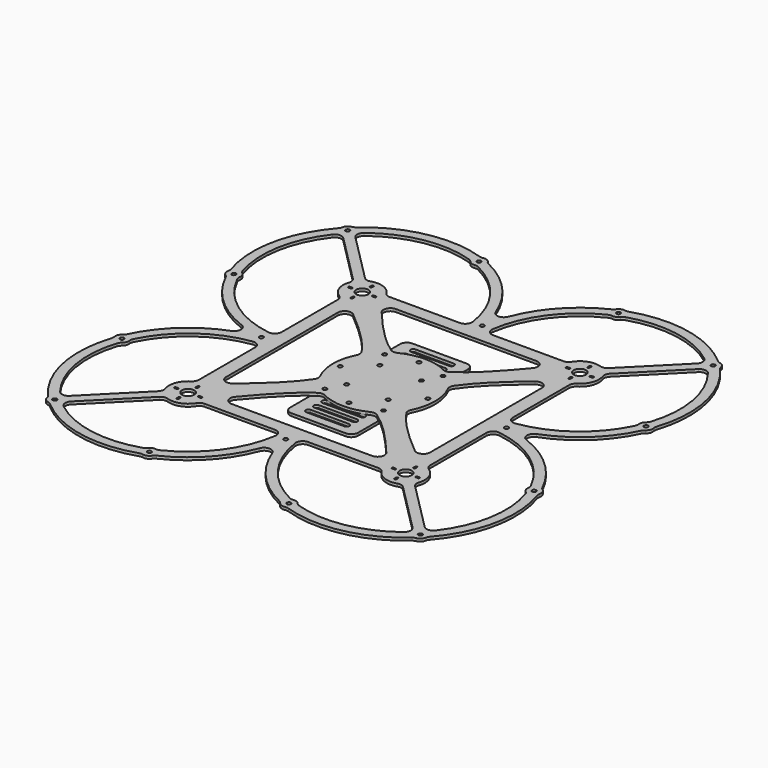
from build123d import *

# Parameters (mm, degrees)
F0_R     = 1.5
F0_R_2   = 4.5
F1_DEPTH = 2
F3_DEPTH = 2
F4_D     = 3
F4_DEPTH = 2.001
F5_D     = 3


with BuildPart() as f1:
    # F0 (on Top) → F1 (new body)
    with BuildSketch(Plane.XY):
        with BuildLine():
            ThreePointArc((-4.6783625728, -108.4060017489), (3e-10, -105.1703496836), (4.6783625734, -108.4060017489))
            ThreePointArc((4.6783625734, -108.4060017489), (20.6623898885, -134.3994303853), (45.1726415046, -152.5762020239))
            ThreePointArc((45.1726415046, -152.5762020239), (46.2648777579, -153.2890175874), (47.1356036045, -154.2600595848))
            ThreePointArc((47.1356036044, -154.2600595849), (49.3956359115, -156.0747849076), (52.2827571645, -156.3307241522))
            ThreePointArc((52.2827571645, -156.3307241521), (53.5833623617, -156.2331937381), (54.8649423602, -156.4753481681))
            ThreePointArc((54.8649423602, -156.4753481681), (96.0251691017, -158.888807541), (132.9814512388, -140.6070608478))
            ThreePointArc((132.9814512388, -140.6070608478), (134.0669737734, -139.8840623088), (135.3025491662, -139.4664027472))
            ThreePointArc((135.3025491663, -139.4664027473), (137.8609824083, -138.1042744963), (139.2338336739, -135.5515791701))
            ThreePointArc((139.2338336738, -135.55157917), (139.6566739459, -134.317767124), (140.3842208964, -133.235287796))
            ThreePointArc((140.3842208964, -133.235287796), (158.8415006809, -96.2563147842), (156.517113249, -54.992373563))
            ThreePointArc((156.517113249, -54.992373563), (156.2770940729, -53.7103919501), (156.3767909625, -52.4099510284))
            ThreePointArc((156.3767909626, -52.4099510283), (156.1256615791, -49.5224074254), (154.3147036453, -47.2593551971))
            ThreePointArc((154.3147036452, -47.2593551972), (153.3451134923, -46.3870129501), (152.6341184177, -45.2935907697))
            ThreePointArc((152.6341184177, -45.2935907697), (134.4488352599, -20.7077210859), (108.4060017484, -4.6783625732))
            ThreePointArc((108.4060017484, -4.6783625732), (105.1703496824, -2e-10), (108.4060017477, 4.6783625732))
            ThreePointArc((108.4060017484, 4.6783625735), (134.4488352601, 20.7077210863), (152.634118418, 45.2935907703))
            ThreePointArc((152.634118418, 45.2935907703), (153.3451134926, 46.3870129507), (154.3147036455, 47.2593551978))
            ThreePointArc((154.3147036455, 47.2593551978), (156.1256615793, 49.5224074261), (156.3767909627, 52.409951029))
            ThreePointArc((156.3767909627, 52.409951029), (156.2770940731, 53.7103919508), (156.5171132493, 54.9923735636))
            ThreePointArc((156.5171132493, 54.9923735636), (158.8415006809, 96.256314785), (140.3842208962, 133.2352877967))
            ThreePointArc((140.3842208962, 133.2352877967), (139.6566739457, 134.3177671247), (139.2338336737, 135.5515791707))
            ThreePointArc((139.2338336737, 135.5515791707), (137.8609824081, 138.1042744969), (135.3025491661, 139.4664027479))
            ThreePointArc((135.3025491661, 139.4664027479), (134.0669737732, 139.8840623095), (132.9814512386, 140.6070608485))
            ThreePointArc((132.9814512386, 140.6070608485), (96.0251691014, 158.8888075416), (54.8649423599, 156.4753481684))
            ThreePointArc((54.8649423599, 156.4753481684), (53.5833623613, 156.2331937384), (52.2827571641, 156.3307241524))
            ThreePointArc((52.2827571641, 156.3307241524), (49.3956359112, 156.0747849078), (47.1356036041, 154.2600595851))
            ThreePointArc((47.1356036041, 154.2600595851), (46.2648777575, 153.2890175877), (45.1726415042, 152.5762020242))
            ThreePointArc((45.1726415042, 152.5762020242), (20.6623898881, 134.3994303854), (4.6783625731, 108.4060017488))
            ThreePointArc((4.6783625731, 108.4060017488), (0, 105.1703496833), (-4.6783625732, 108.4060017486))
            ThreePointArc((-4.6783625731, 108.4060017484), (-20.6623898882, 134.3994303851), (-45.1726415045, 152.576202024))
            ThreePointArc((-45.1726415045, 152.576202024), (-46.2648777578, 153.2890175875), (-47.1356036044, 154.2600595849))
            ThreePointArc((-47.1356036044, 154.2600595849), (-49.3956359115, 156.0747849076), (-52.2827571644, 156.3307241522))
            ThreePointArc((-52.2827571644, 156.3307241522), (-53.5833623617, 156.2331937382), (-54.8649423602, 156.4753481682))
            ThreePointArc((-54.8649423602, 156.4753481682), (-96.0251691017, 158.8888075411), (-132.9814512389, 140.6070608479))
            ThreePointArc((-132.9814512389, 140.6070608479), (-134.0669737735, 139.8840623089), (-135.3025491663, 139.4664027473))
            ThreePointArc((-135.3025491663, 139.4664027473), (-137.8609824083, 138.1042744963), (-139.2338336739, 135.5515791701))
            ThreePointArc((-139.2338336739, 135.5515791701), (-139.656673946, 134.317767124), (-140.3842208964, 133.2352877961))
            ThreePointArc((-140.3842208964, 133.2352877961), (-158.841500681, 96.2563147843), (-156.5171132492, 54.9923735629))
            ThreePointArc((-156.5171132492, 54.9923735629), (-156.277094073, 53.7103919501), (-156.3767909626, 52.4099510283))
            ThreePointArc((-156.3767909626, 52.4099510283), (-156.1256615791, 49.5224074254), (-154.3147036453, 47.2593551971))
            ThreePointArc((-154.3147036453, 47.2593551971), (-153.3451134924, 46.38701295), (-152.6341184178, 45.2935907696))
            ThreePointArc((-152.6341184178, 45.2935907696), (-134.44883526, 20.7077210858), (-108.4060017484, 4.6783625731))
            ThreePointArc((-108.4060017484, 4.6783625731), (-105.1703496831, 0), (-108.4060017484, -4.6783625731))
            ThreePointArc((-108.4060017484, -4.6783625731), (-134.4488352601, -20.7077210859), (-152.6341184181, -45.2935907699))
            ThreePointArc((-152.6341184181, -45.2935907699), (-153.3451134927, -46.3870129503), (-154.3147036456, -47.2593551973))
            ThreePointArc((-154.3147036453, -47.2593551971), (-156.1256615791, -49.5224074254), (-156.3767909626, -52.4099510283))
            ThreePointArc((-156.3767909629, -52.4099510286), (-156.2770940733, -53.7103919503), (-156.5171132495, -54.9923735632))
            ThreePointArc((-156.5171132495, -54.9923735632), (-158.8415006814, -96.2563147847), (-140.3842208967, -133.2352877966))
            ThreePointArc((-140.3842208967, -133.2352877966), (-139.6566739462, -134.3177671246), (-139.2338336742, -135.5515791707))
            ThreePointArc((-139.2338336739, -135.5515791701), (-137.8609824083, -138.1042744963), (-135.3025491663, -139.4664027473))
            ThreePointArc((-135.3025491665, -139.4664027479), (-134.0669737737, -139.8840623095), (-132.9814512391, -140.6070608485))
            ThreePointArc((-132.9814512391, -140.6070608485), (-96.0251691018, -158.8888075418), (-54.8649423601, -156.4753481689))
            ThreePointArc((-54.8649423601, -156.4753481689), (-53.5833623616, -156.2331937389), (-52.2827571643, -156.3307241529))
            ThreePointArc((-52.2827571644, -156.3307241522), (-49.3956359115, -156.0747849076), (-47.1356036044, -154.2600595849))
            ThreePointArc((-47.1356036043, -154.2600595856), (-46.2648777577, -153.2890175882), (-45.1726415044, -152.5762020247))
            ThreePointArc((-45.1726415044, -152.5762020247), (-20.662389888, -134.3994303857), (-4.6783625728, -108.4060017489))
        make_face()
        with Locations((-134.3328737249, -134.5613309295)):
            Circle(F0_R, mode=Mode.SUBTRACT)
        with Locations((-51.261755673, -151.4360785108)):
            Circle(F0_R, mode=Mode.SUBTRACT)
        with BuildLine():
            Line((-63.8445055783, -85.0000000006), (-12.2338580112, -85.0000000003))
            ThreePointArc((-12.2338580112, -85.0000000003), (-8.4490439447, -86.7327102241), (-7.2874242894, -90.7299270076))
            ThreePointArc((-7.2874242894, -90.7299270076), (-20.659248064, -123.3696340744), (-47.697444438, -146.0211701219))
            ThreePointArc((-47.697444438, -146.0211701219), (-49.1034491785, -146.4668977043), (-50.578326435, -146.4830062853))
            ThreePointArc((-50.5783264353, -146.4830062847), (-53.1278754345, -146.797372114), (-55.1848415227, -148.3361757032))
            ThreePointArc((-55.1848415226, -148.3361757039), (-56.2599847867, -149.345922885), (-57.5829585673, -149.9980446406))
            ThreePointArc((-57.5829585673, -149.9980446406), (-92.7749506491, -152.3812865043), (-125.0248290937, -138.0948772713))
            ThreePointArc((-125.0248290937, -138.0948772713), (-126.9516515101, -134.4630557491), (-125.504859117, -130.6147361204))
            Line((-125.504859117, -130.6147361204), (-89.5414765934, -94.5001358666))
            ThreePointArc((-89.5414765934, -94.5001358666), (-87.1537232514, -93.1635209665), (-84.4199717038, -93.2839696686))
            ThreePointArc((-84.4199717038, -93.2839696686), (-75.230169782, -93.1623979469), (-68.0959514787, -87.3684210532))
            ThreePointArc((-68.0959514787, -87.3684210532), (-66.2778268953, -85.6320545604), (-63.8445055783, -85.0000000006))
        make_face(mode=Mode.SUBTRACT)
        with BuildLine():
            ThreePointArc((-79.2499999996, -89.4999999999), (-79.9999999996, -90.2499999999), (-80.7499999996, -89.4999999999))
            Line((-80.7499999996, -89.4999999999), (-80.7499999996, -87.9999999999))
            ThreePointArc((-80.7499999996, -87.9999999999), (-79.9999999996, -87.2499999999), (-79.2499999996, -87.9999999999))
            Line((-79.2499999996, -87.9999999999), (-79.2499999996, -89.4999999999))
        make_face(mode=Mode.SUBTRACT)
        with Locations((-151.4838529462, -51.3807972166)):
            Circle(F0_R, mode=Mode.SUBTRACT)
        with BuildLine():
            ThreePointArc((-85.0000000002, -63.8445055787), (-85.63205456, -66.2778268956), (-87.3684210528, -68.095951479))
            ThreePointArc((-87.3684210528, -68.095951479), (-93.164159415, -75.2350333787), (-93.2806998405, -84.4297868752))
            ThreePointArc((-93.2806998405, -84.4297868752), (-93.156247777, -87.1550368598), (-94.4808633594, -89.5399622996))
            Line((-94.4808633594, -89.5399622996), (-130.4597965629, -125.6701786202))
            ThreePointArc((-130.4597965629, -125.6701786202), (-134.3041683835, -127.1329757672), (-137.9445459786, -125.2181334358))
            ThreePointArc((-137.9445459785, -125.2181334359), (-152.3491388585, -92.9557750247), (-150.035290906, -57.6995957941))
            ThreePointArc((-150.035290906, -57.6995957941), (-149.3853739289, -56.3755375132), (-148.3774191744, -55.2987136553))
            ThreePointArc((-148.3774191741, -55.2987136551), (-146.8420443134, -53.2391870077), (-146.5319260821, -50.6891178603))
            ThreePointArc((-146.5319260824, -50.6891178605), (-146.5182744455, -49.214215816), (-146.0748896721, -47.8074705118))
            ThreePointArc((-146.0748896721, -47.8074705118), (-123.419045392, -20.6953922764), (-90.7299270074, -7.2874242898))
            ThreePointArc((-90.7299270074, -7.2874242898), (-86.7327102239, -8.4490439451), (-85.0000000001, -12.2338580116))
            Line((-85.0000000001, -12.2338580116), (-85.0000000002, -63.8445055787))
        make_face(mode=Mode.SUBTRACT)
        with BuildLine():
            ThreePointArc((-87.9999999996, -79.2499999999), (-87.2499999996, -79.9999999999), (-87.9999999996, -80.7499999999))
            Line((-87.9999999996, -80.7499999999), (-89.4999999996, -80.75))
            ThreePointArc((-89.4999999996, -80.75), (-90.2499999996, -80), (-89.4999999996, -79.25))
            Line((-89.4999999996, -79.25), (-87.9999999996, -79.2499999999))
        make_face(mode=Mode.SUBTRACT)
        with Locations((-80, -80.0000000004)):
            Circle(F0_R_2, mode=Mode.SUBTRACT)
        with BuildLine():
            ThreePointArc((-71.9999999996, -80.7499999998), (-72.7499999996, -79.9999999998), (-71.9999999996, -79.2499999998))
            Line((-71.9999999996, -79.2499999998), (-70.4999999996, -79.2499999998))
            ThreePointArc((-70.4999999996, -79.2499999998), (-69.7499999996, -79.9999999998), (-70.4999999996, -80.7499999998))
            Line((-70.4999999996, -80.7499999998), (-71.9999999996, -80.7499999998))
        make_face(mode=Mode.SUBTRACT)
        with BuildLine():
            ThreePointArc((-79.2499999997, -71.9999999999), (-79.9999999997, -72.7499999999), (-80.7499999997, -71.9999999999))
            Line((-80.7499999997, -71.9999999999), (-80.7499999997, -70.4999999999))
            ThreePointArc((-80.7499999997, -70.4999999999), (-79.9999999997, -69.7499999999), (-79.2499999997, -70.4999999999))
            Line((-79.2499999997, -70.4999999999), (-79.2499999997, -71.9999999999))
        make_face(mode=Mode.SUBTRACT)
        with Locations((51.261755673, -151.4360785108)):
            Circle(F0_R, mode=Mode.SUBTRACT)
        with Locations((4e-10, -90.3351748412)):
            Circle(F0_R, mode=Mode.SUBTRACT)
        with BuildLine():
            Line((12.2338580118, -85.0000000002), (63.8445055786, -85))
            ThreePointArc((63.8445055786, -85), (66.2778268956, -85.6320545598), (68.095951479, -87.3684210526))
            ThreePointArc((68.095951479, -87.3684210526), (75.230169782, -93.1623979461), (84.4199717034, -93.283969668))
            ThreePointArc((84.4199717034, -93.283969668), (87.1537232509, -93.1635209659), (89.5414765929, -94.500135866))
            Line((89.5414765929, -94.500135866), (125.5048591164, -130.6147361197))
            ThreePointArc((125.5048591164, -130.6147361197), (126.9516515096, -134.4630557483), (125.0248290934, -138.0948772705))
            ThreePointArc((125.0248290934, -138.0948772705), (92.774950649, -152.3812865033), (57.5829585674, -149.9980446396))
            ThreePointArc((57.5829585674, -149.9980446396), (56.2599847868, -149.3459228841), (55.1848415227, -148.336175703))
            ThreePointArc((55.1848415227, -148.3361757032), (53.1278754345, -146.797372114), (50.5783264353, -146.4830062847))
            ThreePointArc((50.5783264354, -146.4830062845), (49.1034491789, -146.4668977035), (47.6974444384, -146.021170121))
            ThreePointArc((47.6974444384, -146.021170121), (20.6592480646, -123.3696340739), (7.2874242901, -90.7299270075))
            ThreePointArc((7.2874242901, -90.7299270075), (8.4490439453, -86.732710224), (12.2338580118, -85.0000000002))
        make_face(mode=Mode.SUBTRACT)
        with BuildLine():
            Line((79.2500000004, -89.4999999995), (79.2500000004, -87.9999999995))
            ThreePointArc((79.2500000004, -87.9999999995), (80.0000000004, -87.2499999995), (80.7500000004, -87.9999999995))
            Line((80.7500000004, -87.9999999995), (80.7500000004, -89.4999999995))
            ThreePointArc((80.7500000004, -89.4999999995), (80.0000000004, -90.2499999995), (79.2500000004, -89.4999999995))
        make_face(mode=Mode.SUBTRACT)
        with Locations((134.3328737249, -134.5613309295)):
            Circle(F0_R, mode=Mode.SUBTRACT)
        with BuildLine():
            add(Edge.make_bspline(
                [(-21.8118215176, -33.8721360964), (-14.5412143451, -28.9488980864), (-7.2706071343, -25.9999999845), (7.65e-08, -26)],
                knots=[0.3347589279, 0.3347589279, 0.3347589279, 0.3347589279, 0.5, 0.5, 0.5, 0.5], degree=3))
            add(Edge.make_bspline(
                [(7.65e-08, -26), (7.2706072364, -26.0000000155), (14.5412143964, -28.948898107), (21.8118215577, -33.8721361171)],
                knots=[0.5, 0.5, 0.5, 0.5, 0.6652410721, 0.6652410721, 0.6652410721, 0.6652410721], degree=3))
            add(Edge.make_bspline(
                [(21.8118215178, -33.8721360963), (33.0610814435, -41.4894894667), (44.3103413693, -53.8332210309), (55.5596012951, -67.2936601505)],
                knots=[0.6652410721, 0.6652410721, 0.6652410721, 0.6652410721, 0.9209060704, 0.9209060704, 0.9209060704, 0.9209060704], degree=3))
            ThreePointArc((55.5596012951, -67.2936601505), (56.2524587842, -72.6175812561), (51.7230162552, -75.5))
            Line((51.7230162552, -75.5), (-51.7230162547, -75.5000000003))
            ThreePointArc((-51.7230162547, -75.5000000003), (-56.2524587837, -72.6175812564), (-55.5596012947, -67.2936601507))
            add(Edge.make_bspline(
                [(-55.5596012947, -67.2936601507), (-44.310341369, -53.8332210311), (-33.0610814433, -41.4894894668), (-21.8118215176, -33.8721360964)],
                knots=[0.0790939296, 0.0790939296, 0.0790939296, 0.0790939296, 0.3347589279, 0.3347589279, 0.3347589279, 0.3347589279], degree=3))
        make_face(mode=Mode.SUBTRACT)
        with BuildLine():
            Line((70.5000000004, -79.2499999995), (72.0000000004, -79.2499999995))
            ThreePointArc((72.0000000004, -79.2499999995), (72.7500000004, -79.9999999995), (72.0000000004, -80.7499999995))
            Line((72.0000000004, -80.7499999995), (70.5000000004, -80.7499999995))
            ThreePointArc((70.5000000004, -80.7499999995), (69.7500000004, -79.9999999995), (70.5000000004, -79.2499999995))
        make_face(mode=Mode.SUBTRACT)
        with Locations((80, -80)):
            Circle(F0_R_2, mode=Mode.SUBTRACT)
        with BuildLine():
            ThreePointArc((80.7500000004, -71.9999999995), (80.0000000004, -72.7499999995), (79.2500000004, -71.9999999995))
            Line((79.2500000004, -71.9999999995), (79.2500000004, -70.4999999995))
            ThreePointArc((79.2500000004, -70.4999999995), (80.0000000004, -69.7499999995), (80.7500000004, -70.4999999995))
            Line((80.7500000004, -70.4999999995), (80.7500000004, -71.9999999995))
        make_face(mode=Mode.SUBTRACT)
        with BuildLine():
            add(Edge.make_bspline(
                [(33.8663150036, -21.8197185294), (28.9467838534, -14.548575325), (25.9999990678, -7.2776728311), (25.9999990322, -0.0072165863)],
                knots=[0.3346551775, 0.3346551775, 0.3346551775, 0.3346551775, 0.4998909766, 0.4998909766, 0.4998909766, 0.4998909766], degree=3))
            add(Edge.make_bspline(
                [(25.9999990322, -0.0072165863), (25.9999990322, -0.0048110575), (26.0009742814, 7.2678904272), (28.9508771882, 14.540145319), (33.87301354, 21.8097056412)],
                knots=[0.4998909766, 0.4998909766, 0.4998909766, 0.4998909766, 0.4999456471, 0.6651778067, 0.6651778067, 0.6651778067, 0.6651778067], degree=3))
            add(Edge.make_bspline(
                [(33.87301354, 21.8097056412), (41.3952497644, 32.9193836512), (53.5259879584, 44.0283862504), (66.7895824295, 55.137274203)],
                knots=[0.6651778067, 0.6651778067, 0.6651778067, 0.6651778067, 0.9176932284, 0.9176932284, 0.9176932284, 0.9176932284], degree=3))
            ThreePointArc((66.7895824295, 55.137274203), (72.1151851744, 55.8346983966), (75.0000273883, 51.3041211152))
            Line((75.0000273883, 51.3041211152), (74.9999753624, -51.3429242195))
            ThreePointArc((74.9999753624, -51.3429242195), (72.1142737789, -55.8738975411), (66.7880804223, -55.1748573441))
            add(Edge.make_bspline(
                [(66.7880804223, -55.1748573441), (53.5232646354, -44.0564048176), (41.3886054554, -32.9377802776), (33.8663150036, -21.8197185294)],
                knots=[0.0819986465, 0.0819986465, 0.0819986465, 0.0819986465, 0.3346551775, 0.3346551775, 0.3346551775, 0.3346551775], degree=3))
        make_face(mode=Mode.SUBTRACT)
        with BuildLine():
            Line((88.0000000004, -79.2499999995), (89.5000000004, -79.2499999995))
            ThreePointArc((89.5000000004, -79.2499999995), (90.2500000004, -79.9999999995), (89.5000000004, -80.7499999995))
            Line((89.5000000004, -80.7499999995), (88.0000000004, -80.7499999995))
            ThreePointArc((88.0000000004, -80.7499999995), (87.2500000004, -79.9999999995), (88.0000000004, -79.2499999995))
        make_face(mode=Mode.SUBTRACT)
        with BuildLine():
            ThreePointArc((87.3684210526, -68.095951479), (85.6320545598, -66.2778268956), (85, -63.8445055786))
            Line((85, -63.8445055786), (85, -12.2338580112))
            ThreePointArc((85, -12.2338580112), (86.7327102238, -8.4490439446), (90.7299270073, -7.2874242894))
            ThreePointArc((90.7299270073, -7.2874242894), (123.4190453919, -20.6953922759), (146.0748896721, -47.8074705114))
            ThreePointArc((146.0748896721, -47.8074705114), (146.5182744455, -49.2142158156), (146.5319260824, -50.6891178601))
            ThreePointArc((146.5319260821, -50.6891178603), (146.8420443134, -53.2391870077), (148.3774191741, -55.298713655))
            ThreePointArc((148.3774191744, -55.2987136549), (149.3853739289, -56.3755375129), (150.035290906, -57.6995957937))
            ThreePointArc((150.035290906, -57.6995957937), (152.3491388585, -92.9557750243), (137.9445459785, -125.2181334356))
            ThreePointArc((137.9445459785, -125.2181334356), (134.3041683835, -127.132975767), (130.4597965628, -125.67017862))
            Line((130.4597965628, -125.67017862), (94.4808633591, -89.5399622991))
            ThreePointArc((94.4808633591, -89.5399622991), (93.1562477767, -87.1550368593), (93.2806998402, -84.4297868747))
            ThreePointArc((93.2806998402, -84.4297868747), (93.1641594147, -75.2350333784), (87.3684210526, -68.095951479))
        make_face(mode=Mode.SUBTRACT)
        with Locations((151.4838529462, -51.3807972166)):
            Circle(F0_R, mode=Mode.SUBTRACT)
        with Locations((-90.0851748436, 0)):
            Circle(F0_R, mode=Mode.SUBTRACT)
        with Locations((-151.4838529462, 51.3807972166)):
            Circle(F0_R, mode=Mode.SUBTRACT)
        with BuildLine():
            Line((-85, 63.8445055786), (-85, 12.2338580115))
            ThreePointArc((-85, 12.2338580115), (-86.7327102238, 8.449043945), (-90.7299270073, 7.2874242898))
            ThreePointArc((-90.7299270073, 7.2874242898), (-123.4190453917, 20.6953922762), (-146.0748896718, 47.8074705116))
            ThreePointArc((-146.0748896718, 47.8074705116), (-146.5182744452, 49.2142158157), (-146.5319260821, 50.6891178603))
            ThreePointArc((-146.5319260821, 50.6891178603), (-146.8420443134, 53.2391870077), (-148.3774191741, 55.2987136551))
            ThreePointArc((-148.3774191741, 55.2987136551), (-149.3853739286, 56.375537513), (-150.0352909057, 57.6995957938))
            ThreePointArc((-150.0352909057, 57.6995957938), (-152.3491388582, 92.9557750243), (-137.9445459782, 125.2181334353))
            ThreePointArc((-137.9445459782, 125.2181334353), (-134.3041683832, 127.1329757667), (-130.4597965625, 125.6701786198))
            Line((-130.4597965625, 125.6701786198), (-94.4808633591, 89.5399622991))
            ThreePointArc((-94.4808633591, 89.5399622991), (-93.1562477767, 87.1550368593), (-93.2806998402, 84.4297868747))
            ThreePointArc((-93.2806998402, 84.4297868747), (-93.1641594147, 75.2350333784), (-87.3684210526, 68.095951479))
            ThreePointArc((-87.3684210526, 68.095951479), (-85.6320545598, 66.2778268956), (-85, 63.8445055786))
        make_face(mode=Mode.SUBTRACT)
        with BuildLine():
            Line((-89.5, 80.75), (-88, 80.75))
            ThreePointArc((-88, 80.75), (-87.25, 80), (-88, 79.25))
            Line((-88, 79.25), (-89.5, 79.25))
            ThreePointArc((-89.5, 79.25), (-90.25, 80), (-89.5, 80.75))
        make_face(mode=Mode.SUBTRACT)
        with BuildLine():
            add(Edge.make_bspline(
                [(-33.8721360963, 21.8118215178), (-28.9488980863, 14.5412143452), (-26.0000000096, 7.2706071963), (-26, 4.74e-08)],
                knots=[0.3347589279, 0.3347589279, 0.3347589279, 0.3347589279, 0.5, 0.5, 0.5, 0.5], degree=3))
            add(Edge.make_bspline(
                [(-26, 4.74e-08), (-25.9999999904, -7.2706071331), (-28.9488980734, -14.5412143135), (-33.8721360834, -21.811821493)],
                knots=[0.5, 0.5, 0.5, 0.5, 0.6652410721, 0.6652410721, 0.6652410721, 0.6652410721], degree=3))
            add(Edge.make_bspline(
                [(-33.8721360963, -21.8118215178), (-41.3943179444, -32.9205327334), (-53.5255126569, -44.029243949), (-66.7896643299, -55.1379551646)],
                knots=[0.6652410721, 0.6652410721, 0.6652410721, 0.6652410721, 0.9177117815, 0.9177117815, 0.9177117815, 0.9177117815], degree=3))
            ThreePointArc((-66.7896643299, -55.1379551646), (-72.1152212253, -55.835258214), (-75.0000000043, -51.3047130828))
            Line((-75.0000000043, -51.3047130828), (-75.000000004, 51.3047130826))
            ThreePointArc((-75.000000004, 51.3047130826), (-72.1152212251, 55.8352582138), (-66.7896643296, 55.1379551644))
            add(Edge.make_bspline(
                [(-66.7896643296, 55.1379551644), (-53.5255126568, 44.0292439489), (-41.3943179444, 32.9205327333), (-33.8721360963, 21.8118215178)],
                knots=[0.0822882185, 0.0822882185, 0.0822882185, 0.0822882185, 0.3347589279, 0.3347589279, 0.3347589279, 0.3347589279], degree=3))
        make_face(mode=Mode.SUBTRACT)
        with BuildLine():
            Line((-80.75, 70.5), (-80.75, 72))
            ThreePointArc((-80.75, 72), (-80, 72.75), (-79.25, 72))
            Line((-79.25, 72), (-79.25, 70.5))
            ThreePointArc((-79.25, 70.5), (-80, 69.75), (-80.75, 70.5))
        make_face(mode=Mode.SUBTRACT)
        with Locations((-80, 80)):
            Circle(F0_R_2, mode=Mode.SUBTRACT)
        with BuildLine():
            Line((-70.5, 79.25), (-72, 79.25))
            ThreePointArc((-72, 79.25), (-72.75, 80), (-72, 80.75))
            Line((-72, 80.75), (-70.5, 80.75))
            ThreePointArc((-70.5, 80.75), (-69.75, 80), (-70.5, 79.25))
        make_face(mode=Mode.SUBTRACT)
        with Locations((-134.3328737249, 134.5613309295)):
            Circle(F0_R, mode=Mode.SUBTRACT)
        with BuildLine():
            Line((-79.25, 89.5), (-79.25, 88))
            ThreePointArc((-79.25, 88), (-80, 87.25), (-80.75, 88))
            Line((-80.75, 88), (-80.75, 89.5))
            ThreePointArc((-80.75, 89.5), (-80, 90.25), (-79.25, 89.5))
        make_face(mode=Mode.SUBTRACT)
        with BuildLine():
            ThreePointArc((-63.8445055786, 85), (-66.2778268956, 85.6320545598), (-68.095951479, 87.3684210527))
            ThreePointArc((-68.095951479, 87.3684210527), (-75.2301697821, 93.1623979461), (-84.4199717034, 93.283969668))
            ThreePointArc((-84.4199717034, 93.283969668), (-87.153723251, 93.1635209659), (-89.5414765929, 94.500135866))
            Line((-89.5414765929, 94.500135866), (-125.5048591166, 130.6147361199))
            ThreePointArc((-125.5048591166, 130.6147361199), (-126.9516515098, 134.4630557485), (-125.0248290936, 138.0948772707))
            ThreePointArc((-125.0248290936, 138.0948772707), (-92.774950649, 152.3812865036), (-57.5829585674, 149.9980446399))
            ThreePointArc((-57.5829585674, 149.9980446399), (-56.2599847868, 149.3459228844), (-55.1848415227, 148.3361757032))
            ThreePointArc((-55.1848415227, 148.3361757032), (-53.1278754345, 146.797372114), (-50.5783264353, 146.4830062847))
            ThreePointArc((-50.5783264353, 146.4830062847), (-49.1034491788, 146.4668977038), (-47.6974444383, 146.0211701213))
            ThreePointArc((-47.6974444383, 146.0211701213), (-20.6592480643, 123.369634074), (-7.2874242898, 90.7299270073))
            ThreePointArc((-7.2874242898, 90.7299270073), (-8.4490439451, 86.7327102239), (-12.2338580115, 85.0000000002))
            Line((-12.2338580115, 85.0000000002), (-63.8445055786, 85))
        make_face(mode=Mode.SUBTRACT)
        with Locations((-51.261755673, 151.4360785108)):
            Circle(F0_R, mode=Mode.SUBTRACT)
        Polygon((26, -0.0072165863), (26, -26), (1.147e-07, -26), (-26, -26), (-26, 7.1e-08), (-26, 26), (-7.1e-08, 26), (26, 26), align=None, mode=Mode.SUBTRACT)
        with BuildLine():
            add(Edge.make_bspline(
                [(-4.74e-08, 26), (7.2706071331, 25.9999999904), (14.5412143135, 28.9488980734), (21.811821493, 33.8721360834)],
                knots=[0.5, 0.5, 0.5, 0.5, 0.6652410721, 0.6652410721, 0.6652410721, 0.6652410721], degree=3))
            add(Edge.make_bspline(
                [(-21.8118215178, 33.8721360963), (-14.5412143452, 28.9488980863), (-7.2706071963, 26.0000000096), (-4.74e-08, 26)],
                knots=[0.3347589279, 0.3347589279, 0.3347589279, 0.3347589279, 0.5, 0.5, 0.5, 0.5], degree=3))
            add(Edge.make_bspline(
                [(-55.5596012951, 67.2936601505), (-44.3103413693, 53.8332210308), (-33.0610814435, 41.4894894667), (-21.8118215178, 33.8721360963)],
                knots=[0.0790939296, 0.0790939296, 0.0790939296, 0.0790939296, 0.3347589279, 0.3347589279, 0.3347589279, 0.3347589279], degree=3))
            ThreePointArc((-55.5596012951, 67.2936601505), (-56.2524587842, 72.6175812561), (-51.7230162551, 75.5))
            Line((-51.7230162551, 75.5), (51.7230162553, 75.5000000003))
            ThreePointArc((51.7230162553, 75.5000000003), (56.2524587844, 72.6175812564), (55.5596012953, 67.2936601507))
            add(Edge.make_bspline(
                [(21.8118215178, 33.8721360963), (33.0610814436, 41.4894894667), (44.3103413695, 53.833221031), (55.5596012953, 67.2936601507)],
                knots=[0.6652410721, 0.6652410721, 0.6652410721, 0.6652410721, 0.9209060704, 0.9209060704, 0.9209060704, 0.9209060704], degree=3))
        make_face(mode=Mode.SUBTRACT)
        with BuildLine():
            ThreePointArc((79.25, 72.0000000004), (80, 72.7500000004), (80.75, 72.0000000004))
            Line((80.75, 72.0000000004), (80.75, 70.5000000004))
            ThreePointArc((80.75, 70.5000000004), (80, 69.7500000004), (79.25, 70.5000000004))
            Line((79.25, 70.5000000004), (79.25, 72.0000000004))
        make_face(mode=Mode.SUBTRACT)
        with BuildLine():
            ThreePointArc((72, 80.7500000003), (72.75, 80.0000000003), (72, 79.2500000003))
            Line((72, 79.2500000003), (70.5, 79.2500000003))
            ThreePointArc((70.5, 79.2500000003), (69.75, 80.0000000003), (70.5, 80.7500000003))
            Line((70.5, 80.7500000003), (72, 80.7500000003))
        make_face(mode=Mode.SUBTRACT)
        with Locations((80, 80.0000000004)):
            Circle(F0_R_2, mode=Mode.SUBTRACT)
        with Locations((90.085174844, 5e-10)):
            Circle(F0_R, mode=Mode.SUBTRACT)
        with BuildLine():
            ThreePointArc((89.5, 80.7500000004), (90.25, 80.0000000004), (89.5, 79.2500000004))
            Line((89.5, 79.2500000004), (88, 79.2500000004))
            ThreePointArc((88, 79.2500000004), (87.25, 80.0000000004), (88, 80.7500000004))
            Line((88, 80.7500000004), (89.5, 80.7500000004))
        make_face(mode=Mode.SUBTRACT)
        with BuildLine():
            ThreePointArc((85, 63.844505579), (85.6320545598, 66.2778268959), (87.3684210526, 68.0959514793))
            ThreePointArc((87.3684210526, 68.0959514793), (93.1641594147, 75.2350333788), (93.2806998401, 84.4297868751))
            ThreePointArc((93.2806998401, 84.4297868751), (93.1562477767, 87.1550368597), (94.4808633591, 89.5399622995))
            Line((94.4808633591, 89.5399622995), (130.4597965625, 125.6701786201))
            ThreePointArc((130.4597965625, 125.6701786201), (134.3041683832, 127.1329757671), (137.9445459782, 125.2181334357))
            ThreePointArc((137.9445459782, 125.2181334357), (152.3491388582, 92.9557750248), (150.0352909058, 57.6995957945))
            ThreePointArc((150.0352909058, 57.6995957945), (149.3853739287, 56.3755375137), (148.3774191742, 55.2987136557))
            ThreePointArc((148.3774191742, 55.2987136557), (146.8420443135, 53.2391870084), (146.5319260822, 50.6891178609))
            ThreePointArc((146.5319260822, 50.6891178609), (146.5182744454, 49.2142158164), (146.0748896719, 47.8074705122))
            ThreePointArc((146.0748896719, 47.8074705122), (123.4190453919, 20.6953922767), (90.7299270073, 7.2874242901))
            ThreePointArc((90.7299270073, 7.2874242901), (86.7327102238, 8.4490439454), (85, 12.2338580119))
            Line((85, 12.2338580119), (85, 63.844505579))
        make_face(mode=Mode.SUBTRACT)
        with Locations((151.4838529464, 51.3807972172)):
            Circle(F0_R, mode=Mode.SUBTRACT)
        with Locations((0, 90.3351748417)):
            Circle(F0_R, mode=Mode.SUBTRACT)
        with BuildLine():
            ThreePointArc((80.75, 88.0000000004), (80, 87.2500000004), (79.25, 88.0000000004))
            Line((79.25, 88.0000000004), (79.25, 89.5000000004))
            ThreePointArc((79.25, 89.5000000004), (80, 90.2500000004), (80.75, 89.5000000004))
            Line((80.75, 89.5000000004), (80.75, 88.0000000004))
        make_face(mode=Mode.SUBTRACT)
        with BuildLine():
            ThreePointArc((68.095951479, 87.368421053), (66.2778268956, 85.6320545602), (63.8445055786, 85.0000000003))
            Line((63.8445055786, 85.0000000003), (12.2338580115, 85.0000000002))
            ThreePointArc((12.2338580115, 85.0000000002), (8.4490439449, 86.732710224), (7.2874242898, 90.7299270077))
            ThreePointArc((7.2874242898, 90.7299270077), (20.6592480642, 123.3696340742), (47.697444438, 146.0211701215))
            ThreePointArc((47.697444438, 146.0211701215), (49.1034491785, 146.466897704), (50.578326435, 146.4830062849))
            ThreePointArc((50.578326435, 146.4830062849), (53.1278754342, 146.7973721143), (55.1848415223, 148.3361757035))
            ThreePointArc((55.1848415223, 148.3361757035), (56.2599847865, 149.3459228846), (57.582958567, 149.9980446401))
            ThreePointArc((57.582958567, 149.9980446401), (92.7749506489, 152.381286504), (125.0248290935, 138.0948772711))
            ThreePointArc((125.0248290935, 138.0948772711), (126.9516515098, 134.4630557488), (125.5048591166, 130.6147361202))
            Line((125.5048591166, 130.6147361202), (89.5414765929, 94.5001358664))
            ThreePointArc((89.5414765929, 94.5001358664), (87.1537232509, 93.1635209663), (84.4199717034, 93.2839696684))
            ThreePointArc((84.4199717034, 93.2839696684), (75.230169782, 93.1623979465), (68.095951479, 87.368421053))
        make_face(mode=Mode.SUBTRACT)
        with Locations((51.2617556727, 151.436078511)):
            Circle(F0_R, mode=Mode.SUBTRACT)
        with Locations((134.3328737246, 134.5613309301)):
            Circle(F0_R, mode=Mode.SUBTRACT)
        Polygon((1.147e-07, -26), (26, -26), (26, -0.0072165863), (26, 26), (-7.1e-08, 26), (-26, 26), (-26, 7.1e-08), (-26, -26), align=None)
        with Locations((-15.25, -15.25)):
            Circle(F0_R, mode=Mode.SUBTRACT)
        with Locations((15.25, -15.25)):
            Circle(F0_R, mode=Mode.SUBTRACT)
        with Locations((-15.25, 15.25)):
            Circle(F0_R, mode=Mode.SUBTRACT)
        with Locations((15.25, 15.25)):
            Circle(F0_R, mode=Mode.SUBTRACT)
        with BuildLine():
            add(Edge.make_bspline(
                [(25.9999990322, -0.0072165863), (25.9999990322, -0.0048110575), (26.0009742814, 7.2678904272), (28.9508771882, 14.540145319), (33.87301354, 21.8097056412)],
                knots=[0.4998909766, 0.4998909766, 0.4998909766, 0.4998909766, 0.4999456471, 0.6651778067, 0.6651778067, 0.6651778067, 0.6651778067], degree=3))
            add(Edge.make_bspline(
                [(33.8663150036, -21.8197185294), (28.9467838534, -14.548575325), (25.9999990678, -7.2776728311), (25.9999990322, -0.0072165863)],
                knots=[0.3346551775, 0.3346551775, 0.3346551775, 0.3346551775, 0.4998909766, 0.4998909766, 0.4998909766, 0.4998909766], degree=3))
            ThreePointArc((33.8663150036, -21.8197185294), (33.0182203428, -19.3448492461), (33.5360437181, -16.7804581926))
            ThreePointArc((33.5360437181, -16.7804581926), (37.4999996469, -0.0056476076), (33.5410965671, 16.7703561827))
            ThreePointArc((33.5410965671, 16.7703561827), (33.0240531169, 19.3350168644), (33.87301354, 21.8097056412))
        make_face()
        with Locations((32.1965969132, 0)):
            Circle(F0_R, mode=Mode.SUBTRACT)
        with BuildLine():
            add(Edge.make_bspline(
                [(7.65e-08, -26), (7.2706072364, -26.0000000155), (14.5412143964, -28.948898107), (21.8118215577, -33.8721361171)],
                knots=[0.5, 0.5, 0.5, 0.5, 0.6652410721, 0.6652410721, 0.6652410721, 0.6652410721], degree=3))
            add(Edge.make_bspline(
                [(-21.8118215176, -33.8721360964), (-14.5412143451, -28.9488980864), (-7.2706071343, -25.9999999845), (7.65e-08, -26)],
                knots=[0.3347589279, 0.3347589279, 0.3347589279, 0.3347589279, 0.5, 0.5, 0.5, 0.5], degree=3))
            ThreePointArc((-21.8118215176, -33.8721360964), (-19.336942988, -33.0230694214), (-16.7720877967, -33.5402307141))
            ThreePointArc((-16.7720877967, -33.5402307141), (1e-10, -37.5000000722), (16.7720877969, -33.540230714))
            ThreePointArc((16.7720877969, -33.540230714), (19.3369429881, -33.0230694213), (21.8118215178, -33.8721360963))
        make_face()
        with Locations((0, -32.2011839358)):
            Circle(F0_R, mode=Mode.SUBTRACT)
        with BuildLine():
            add(Edge.make_bspline(
                [(-26, 4.74e-08), (-25.9999999904, -7.2706071331), (-28.9488980734, -14.5412143135), (-33.8721360834, -21.811821493)],
                knots=[0.5, 0.5, 0.5, 0.5, 0.6652410721, 0.6652410721, 0.6652410721, 0.6652410721], degree=3))
            add(Edge.make_bspline(
                [(-33.8721360963, 21.8118215178), (-28.9488980863, 14.5412143452), (-26.0000000096, 7.2706071963), (-26, 4.74e-08)],
                knots=[0.3347589279, 0.3347589279, 0.3347589279, 0.3347589279, 0.5, 0.5, 0.5, 0.5], degree=3))
            ThreePointArc((-33.8721360963, 21.8118215178), (-33.0230694213, 19.3369429881), (-33.540230714, 16.7720877968))
            ThreePointArc((-33.540230714, 16.7720877968), (-37.5000000722, 0), (-33.540230714, -16.7720877968))
            ThreePointArc((-33.540230714, -16.7720877968), (-33.0230694213, -19.3369429881), (-33.8721360963, -21.8118215178))
        make_face()
        with Locations((-32.1965969128, -1e-10)):
            Circle(F0_R, mode=Mode.SUBTRACT)
        with BuildLine():
            add(Edge.make_bspline(
                [(-21.8118215178, 33.8721360963), (-14.5412143452, 28.9488980863), (-7.2706071963, 26.0000000096), (-4.74e-08, 26)],
                knots=[0.3347589279, 0.3347589279, 0.3347589279, 0.3347589279, 0.5, 0.5, 0.5, 0.5], degree=3))
            add(Edge.make_bspline(
                [(-4.74e-08, 26), (7.2706071331, 25.9999999904), (14.5412143135, 28.9488980734), (21.811821493, 33.8721360834)],
                knots=[0.5, 0.5, 0.5, 0.5, 0.6652410721, 0.6652410721, 0.6652410721, 0.6652410721], degree=3))
            ThreePointArc((21.8118215178, 33.8721360963), (19.3369429881, 33.0230694213), (16.7720877968, 33.540230714))
            ThreePointArc((16.7720877968, 33.540230714), (0, 37.5000000722), (-16.7720877968, 33.540230714))
            ThreePointArc((-16.7720877968, 33.540230714), (-19.3369429881, 33.0230694213), (-21.8118215178, 33.8721360963))
        make_face()
        with Locations((0, 32.2011839358)):
            Circle(F0_R, mode=Mode.SUBTRACT)
    extrude(amount=F1_DEPTH)

    # F5 (through all)
    with Locations(Plane(origin=(0, 0, 0), x_dir=(1, 0, 0), z_dir=(0, 0, -1))):
        with Locations((-21.5, 27.4696089327), (21.5, 27.4696089327), (21.5, -27.4696089327), (-21.5, -27.4696089327)):
            Hole(F5_D / 2)


with BuildPart() as f3:
    # F2 (on face) → F3 (new body)
    with BuildSketch(Plane(origin=(0, 0, 0), x_dir=(1, 0, 0), z_dir=(0, 0, -1))):
        with BuildLine():
            Line((-20, -51), (20, -51))
            ThreePointArc((20, -51), (23.5355339059, -49.5355339059), (25, -46))
            Line((25, -46), (25, 0))
            Line((25, 0), (25, 46))
            Line((25, 46), (25, 55))
            ThreePointArc((25, 55), (23.5355339059, 58.5355339059), (20, 60))
            Line((20, 60), (-20, 60))
            ThreePointArc((-20, 60), (-23.5355339059, 58.5355339059), (-25, 55))
            Line((-25, 55), (-25, 46))
            Line((-25, 46), (-25, 0))
            Line((-25, 0), (-25, -46))
            ThreePointArc((-25, -46), (-23.5355339059, -49.5355339059), (-20, -51))
        make_face()
        with BuildLine():
            Line((-20, 15), (-20, -15))
            ThreePointArc((-20, -15), (-21.5, -16.5), (-23, -15))
            Line((-23, -15), (-23, 15))
            ThreePointArc((-23, 15), (-21.5, 16.5), (-20, 15))
        make_face(mode=Mode.SUBTRACT)
        with BuildLine():
            ThreePointArc((-14.0279019251, -46.4), (-16.0279019251, -44.4), (-14.0279019251, -42.4))
            Line((-14.0279019251, -42.4), (14.0279019251, -42.4))
            ThreePointArc((14.0279019251, -42.4), (16.0279019251, -44.4), (14.0279019251, -46.4))
            Line((14.0279019251, -46.4), (-14.0279019251, -46.4))
        make_face(mode=Mode.SUBTRACT)
        with BuildLine():
            ThreePointArc((14.0279019251, -35), (16.0279019251, -37), (14.0279019251, -39))
            Line((14.0279019251, -39), (-14.0279019251, -39))
            ThreePointArc((-14.0279019251, -39), (-16.0279019251, -37), (-14.0279019251, -35))
            Line((-14.0279019251, -35), (14.0279019251, -35))
        make_face(mode=Mode.SUBTRACT)
        with BuildLine():
            ThreePointArc((-14.0279019251, -31.6), (-16.0279019251, -29.6), (-14.0279019251, -27.6))
            Line((-14.0279019251, -27.6), (14.0279019251, -27.6))
            ThreePointArc((14.0279019251, -27.6), (16.0279019251, -29.6), (14.0279019251, -31.6))
            Line((14.0279019251, -31.6), (-14.0279019251, -31.6))
        make_face(mode=Mode.SUBTRACT)
        with BuildLine():
            ThreePointArc((-14.0279019251, -24.2), (-16.0279019251, -22.2), (-14.0279019251, -20.2))
            Line((-14.0279019251, -20.2), (14.0279019251, -20.2))
            ThreePointArc((14.0279019251, -20.2), (16.0279019251, -22.2), (14.0279019251, -24.2))
            Line((14.0279019251, -24.2), (-14.0279019251, -24.2))
        make_face(mode=Mode.SUBTRACT)
        with BuildLine():
            ThreePointArc((-14.0279019251, -16.8), (-16.0279019251, -14.8), (-14.0279019251, -12.8))
            Line((-14.0279019251, -12.8), (14.0279019251, -12.8))
            ThreePointArc((14.0279019251, -12.8), (16.0279019251, -14.8), (14.0279019251, -16.8))
            Line((14.0279019251, -16.8), (-14.0279019251, -16.8))
        make_face(mode=Mode.SUBTRACT)
        with BuildLine():
            ThreePointArc((-14.0279019251, -9.4), (-16.0279019251, -7.4), (-14.0279019251, -5.4))
            Line((-14.0279019251, -5.4), (14.0279019251, -5.4))
            ThreePointArc((14.0279019251, -5.4), (16.0279019251, -7.4), (14.0279019251, -9.4))
            Line((14.0279019251, -9.4), (-14.0279019251, -9.4))
        make_face(mode=Mode.SUBTRACT)
        with BuildLine():
            Line((14.0279019251, -2), (-14.0279019251, -2))
            ThreePointArc((-14.0279019251, -2), (-16.0279019251, 0), (-14.0279019251, 2))
            Line((-14.0279019251, 2), (14.0279019251, 2))
            ThreePointArc((14.0279019251, 2), (16.0279019251, 0), (14.0279019251, -2))
        make_face(mode=Mode.SUBTRACT)
        with BuildLine():
            Line((23, 15), (23, -15))
            ThreePointArc((23, -15), (21.5, -16.5), (20, -15))
            Line((20, -15), (20, 15))
            ThreePointArc((20, 15), (21.5, 16.5), (23, 15))
        make_face(mode=Mode.SUBTRACT)
        with BuildLine():
            ThreePointArc((-14.0279019251, 5.4), (-16.0279019251, 7.4), (-14.0279019251, 9.4))
            Line((-14.0279019251, 9.4), (14.0279019251, 9.4))
            ThreePointArc((14.0279019251, 9.4), (16.0279019251, 7.4), (14.0279019251, 5.4))
            Line((14.0279019251, 5.4), (-14.0279019251, 5.4))
        make_face(mode=Mode.SUBTRACT)
        with BuildLine():
            ThreePointArc((-14.0279019251, 12.8), (-16.0279019251, 14.8), (-14.0279019251, 16.8))
            Line((-14.0279019251, 16.8), (14.0279019251, 16.8))
            ThreePointArc((14.0279019251, 16.8), (16.0279019251, 14.8), (14.0279019251, 12.8))
            Line((14.0279019251, 12.8), (-14.0279019251, 12.8))
        make_face(mode=Mode.SUBTRACT)
        with BuildLine():
            ThreePointArc((-14.0279019251, 20.2), (-16.0279019251, 22.2), (-14.0279019251, 24.2))
            Line((-14.0279019251, 24.2), (14.0279019251, 24.2))
            ThreePointArc((14.0279019251, 24.2), (16.0279019251, 22.2), (14.0279019251, 20.2))
            Line((14.0279019251, 20.2), (-14.0279019251, 20.2))
        make_face(mode=Mode.SUBTRACT)
        with BuildLine():
            ThreePointArc((-14.0279019251, 27.6), (-16.0279019251, 29.6), (-14.0279019251, 31.6))
            Line((-14.0279019251, 31.6), (14.0279019251, 31.6))
            ThreePointArc((14.0279019251, 31.6), (16.0279019251, 29.6), (14.0279019251, 27.6))
            Line((14.0279019251, 27.6), (-14.0279019251, 27.6))
        make_face(mode=Mode.SUBTRACT)
        with BuildLine():
            ThreePointArc((-14.0279019251, 35), (-16.0279019251, 37), (-14.0279019251, 39))
            Line((-14.0279019251, 39), (14.0279019251, 39))
            ThreePointArc((14.0279019251, 39), (16.0279019251, 37), (14.0279019251, 35))
            Line((14.0279019251, 35), (-14.0279019251, 35))
        make_face(mode=Mode.SUBTRACT)
        with BuildLine():
            ThreePointArc((-14.0279019251, 42.4), (-16.0279019251, 44.4), (-14.0279019251, 46.4))
            Line((-14.0279019251, 46.4), (14.0279019251, 46.4))
            ThreePointArc((14.0279019251, 46.4), (16.0279019251, 44.4), (14.0279019251, 42.4))
            Line((14.0279019251, 42.4), (-14.0279019251, 42.4))
        make_face(mode=Mode.SUBTRACT)
        with BuildLine():
            ThreePointArc((-14.0279019251, 49.8), (-16.0279019251, 51.8), (-14.0279019251, 53.8))
            Line((-14.0279019251, 53.8), (14.0279019251, 53.8))
            ThreePointArc((14.0279019251, 53.8), (16.0279019251, 51.8), (14.0279019251, 49.8))
            Line((14.0279019251, 49.8), (-14.0279019251, 49.8))
        make_face(mode=Mode.SUBTRACT)
    extrude(amount=F3_DEPTH)

    # F4 (through all, one way)
    with BuildSketch(Plane.XY):
        with Locations((-21.5, -27.4696089327), (21.5, -27.4696089327), (-21.5, 27.4696089327), (21.5, 27.4696089327)):
            Circle(F4_D / 2)
    extrude(amount=-F4_DEPTH, mode=Mode.SUBTRACT)


solid = Compound([f1.part, f3.part])
